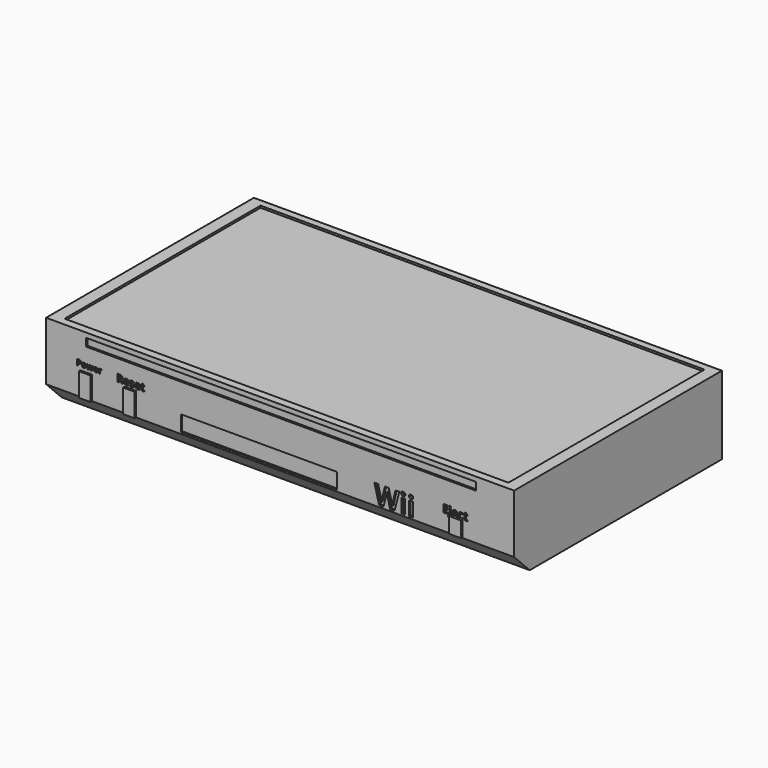
from build123d import *

# Parameters (mm, degrees)
F0_W          = 120
F0_H          = 20
F1_DEPTH      = 66.6
F2_SIZE       = 5
F4_W          = 40
F4_H          = 4
F6_DEPTH      = 0.4
F3_W          = 3
F3_H          = 6
F3_W_2        = 2.9399991035
F7_DEPTH      = 0.5
F9_TEXT_SIZE  = 2.0881390406
F10_DEPTH     = 0.5
F5_TEXT_SIZE  = 6.603775546
F11_DEPTH     = 0.5
F12_TEXT_SIZE = 2.6249999387
F13_DEPTH     = 0.5
F14_W         = 3
F14_H         = 4
F15_DEPTH     = 0.5
F16_W         = 113.8200052083
F16_H         = 62.7900036052
F17_DEPTH     = 0.5
F8_W          = 100
F8_H          = 2
F18_DEPTH     = 0.5
F19_TEXT_SIZE = 2.7266779914
F20_DEPTH     = 0.5
F21_W         = 115.9200035036
F21_H         = 16.8000012636
F22_DEPTH     = 0.5


# Not quite as in the source:
# - Text() gives the source's letters only with a copy of the font that has no kerning and outlines rounded to 1/6400 em; it was checked with that copy


with BuildPart() as f1:
    # F0 (on Front) → F1 (new body)
    with BuildSketch(Plane.XZ):
        with Locations((3.6149969697, 24.5950010046)):
            Rectangle(F0_W, F0_H)
    extrude(amount=-F1_DEPTH)

    # F2
    f2_edges = [f1.edges().sort_by_distance(p)[0] for p in [
        (3.614997, 0, 14.595001),
    ]]
    chamfer(f2_edges, length=F2_SIZE)

    # F4 (on face) → F6 (cut)
    with BuildSketch(Plane.XZ):
        with Locations((-1.8349983543, 22.0550016016)):
            Rectangle(F4_W, F4_H)
    extrude(amount=-F6_DEPTH, mode=Mode.SUBTRACT)

    # F3 (on face) → F7 (join)
    with BuildSketch(Plane.XZ):
        with Locations((-46.0650019944, 22.5950010046)):
            Rectangle(F3_W, F3_H)
        with Locations((-34.7550027072, 22.5950010046)):
            Rectangle(F3_W_2, F3_H)
    extrude(amount=F7_DEPTH)

    # F9 (on face) → F10 (cut)
    with BuildSketch(Plane.XZ):
        with Locations((-48.6460216343, 26.4192447066)):
            Text('Power', F9_TEXT_SIZE, font='Open Sans', font_style=FontStyle.BOLD, text_align=(TextAlign.LEFT, TextAlign.BOTTOM))
    extrude(amount=-F10_DEPTH, mode=Mode.SUBTRACT)

    # F5 (on face) → F11 (cut)
    with BuildSketch(Plane.XZ):
        with Locations((27.7853775769, 20.0589615852)):
            Text('Wii', F5_TEXT_SIZE, font='Open Sans', font_style=FontStyle.BOLD, text_align=(TextAlign.LEFT, TextAlign.BOTTOM))
    extrude(amount=-F11_DEPTH, mode=Mode.SUBTRACT)

    # F12 (on face) → F13 (cut)
    with BuildSketch(Plane.XZ):
        with Locations((-38.3250005543, 26.0624997318)):
            Text('Reset', F12_TEXT_SIZE, font='Open Sans', font_style=FontStyle.BOLD, text_align=(TextAlign.LEFT, TextAlign.BOTTOM))
    extrude(amount=-F13_DEPTH, mode=Mode.SUBTRACT)

    # F14 (on face) → F15 (join)
    with BuildSketch(Plane.XZ):
        with Locations((48.8702871501, 21.7617933154)):
            Rectangle(F14_W, F14_H)
    extrude(amount=F15_DEPTH)

    # F16 (on face) → F17 (cut)
    with BuildSketch(Plane.XY.offset(34.5950010046)):
        with Locations((3.6750007421, 33.3900018595)):
            Rectangle(F16_W, F16_H)
    extrude(amount=-F17_DEPTH, mode=Mode.SUBTRACT)

    # F8 (on face) → F18 (cut)
    with BuildSketch(Plane.XZ):
        with Locations((3.8650006056, 32.3949994743)):
            Rectangle(F8_W, F8_H)
    extrude(amount=-F18_DEPTH, mode=Mode.SUBTRACT)

    # F19 (on face) → F20 (cut)
    with BuildSketch(Plane.XZ):
        with Locations((45.2549979091, 23.7617933154)):
            Text('Eject', F19_TEXT_SIZE, font='Open Sans', font_style=FontStyle.BOLD, text_align=(TextAlign.LEFT, TextAlign.BOTTOM))
    extrude(amount=-F20_DEPTH, mode=Mode.SUBTRACT)

    # F21 (on face) → F22 (cut)
    with BuildSketch(Plane(origin=(0, 66.6, 0), x_dir=(-1, 0, 0), z_dir=(0, 1, 0))):
        with Locations((-3.6750007421, 24.675000459)):
            Rectangle(F21_W, F21_H)
    extrude(amount=-F22_DEPTH, mode=Mode.SUBTRACT)


solid = f1.part
